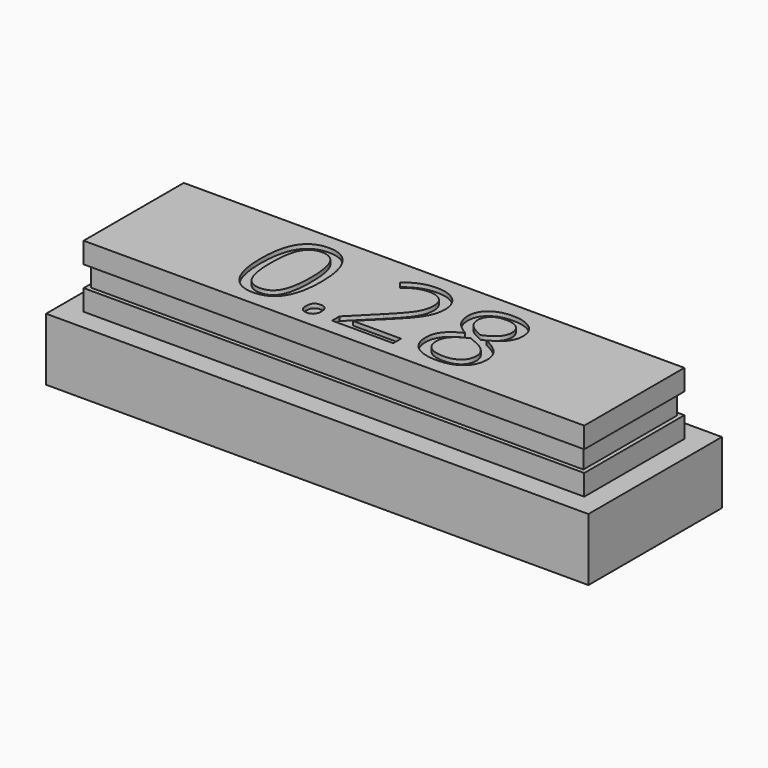
from build123d import *

# Parameters (mm, degrees)
F0_W         = 26
F0_H         = 8
F0_W_2       = 20
F0_H_2       = 2
F1_DEPTH     = 3
F2_W         = 24
F2_H         = 6
F3_DEPTH     = 3
F5_W         = 24
F5_H         = 6
F5_W_2       = 23.6
F5_H_2       = 5.6
F6_DEPTH     = 0.5
F7_W         = 19.44
F7_H         = 1.44
F8_DEPTH     = 3
F9_TEXT_SIZE = 6.25
F10_DEPTH    = 0.2


# Not quite as in the source:
# - Text() gives the source's letters only with a copy of the font that has no kerning and outlines rounded to 1/6400 em; it was checked with that copy


with BuildPart() as f1:
    # F0 (on Top) → F1 (new body)
    with BuildSketch(Plane.XY):
        Rectangle(F0_W, F0_H)
        Rectangle(F0_W_2, F0_H_2, mode=Mode.SUBTRACT)
    extrude(amount=F1_DEPTH)


with BuildPart() as f3:
    # F2 (on face) → F3 (new body)
    with BuildSketch(Plane.XY.offset(3)):
        Rectangle(F2_W, F2_H)
    extrude(amount=F3_DEPTH)

    # F5 (on mid) → F6 (cut, symmetric)
    with BuildSketch(Plane.XY.offset(4.5)):
        Rectangle(F5_W, F5_H)
        Rectangle(F5_W_2, F5_H_2, mode=Mode.SUBTRACT)
    extrude(amount=F6_DEPTH, both=True, mode=Mode.SUBTRACT)

    # F7 (on face) → F8 (join, through all)
    with BuildSketch(Plane(origin=(0, 0, 3), x_dir=(1, 0, 0), z_dir=(0, 0, -1))):
        Rectangle(F7_W, F7_H)
    extrude(amount=F8_DEPTH)

    # F9 (on face) → F10 (cut)
    with BuildSketch(Plane.XY.offset(6)):
        with Locations((-6.232421875, -2.25)):
            Text('0.28', F9_TEXT_SIZE, font='Open Sans', text_align=(TextAlign.LEFT, TextAlign.BOTTOM))
    extrude(amount=-F10_DEPTH, mode=Mode.SUBTRACT)


solid = Compound([f1.part, f3.part])
